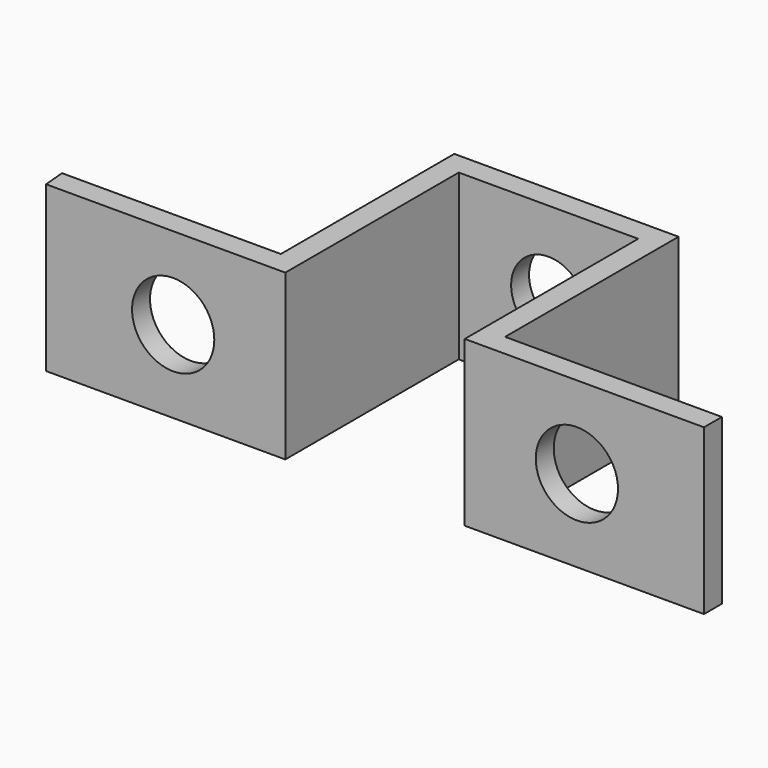
from build123d import *

# Parameters (mm, degrees)
F1_DEPTH = 22
F2_R     = 5
F3_DEPTH = 10
F4_R     = 5.5
F5_DEPTH = 25


# Not quite as in the source:
# - a feature names something its author has since deleted; it is built from what else it names


with BuildPart() as f1:
    # F0 (on Top) → F1 (new body)
    with BuildSketch(Plane.XY):
        Polygon((-15, -15.631636476), (-44.2782626623, -15.631636476), (-44, -18.631636476), (-12, -18.631636476), (-12, 10.368363524), (12, 10.368363524), (12, -18.631636476), (44, -18.631636476), (44, -15.631636476), (15, -15.631636476), (15, 13.368363524), (-15, 13.368363524), align=None)
    extrude(amount=F1_DEPTH)

    # F2 (on face) → F3 (cut)
    with BuildSketch(Plane(origin=(0, 13.368363524, 0), x_dir=(-1, 0, 0), z_dir=(0, 1, 0))):
        with Locations((0, 11)):
            Circle(F2_R)
    extrude(amount=-F3_DEPTH, mode=Mode.SUBTRACT)

    # F4 (on Front) → F5 (cut)
    with BuildSketch(Plane.XZ):
        with Locations((27, 11)):
            Circle(F4_R)
        with Locations((-27, 11)):
            Circle(F4_R)
    extrude(amount=F5_DEPTH, mode=Mode.SUBTRACT)


solid = f1.part
